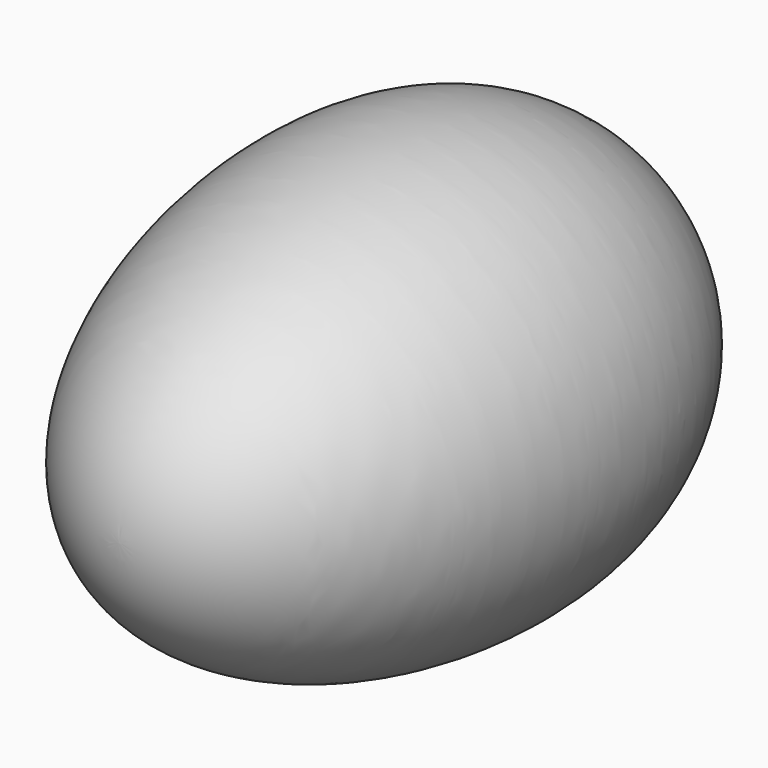
from build123d import *


with BuildPart() as f1:
    # F0 (on Right) → F1 (revolve)
    with BuildSketch(Plane.YZ):
        with BuildLine():
            add(Edge.make_bspline(
                [(-31.7243337631, 0), (-31.6051058471, 18.788035959), (21.7730031814, 37.1740843736), (46.2017537703, 14.2193894453), (45.5741398036, 0)],
                knots=[0, 0, 0, 0, 0.5496852598, 1, 1, 1, 1], degree=3))
            Line((-31.7243337631, 0), (45.5741398036, 0))
        make_face()
    revolve(axis=Axis((0, 0.8879229426, 0), (0, 1, 0)))


solid = f1.part
